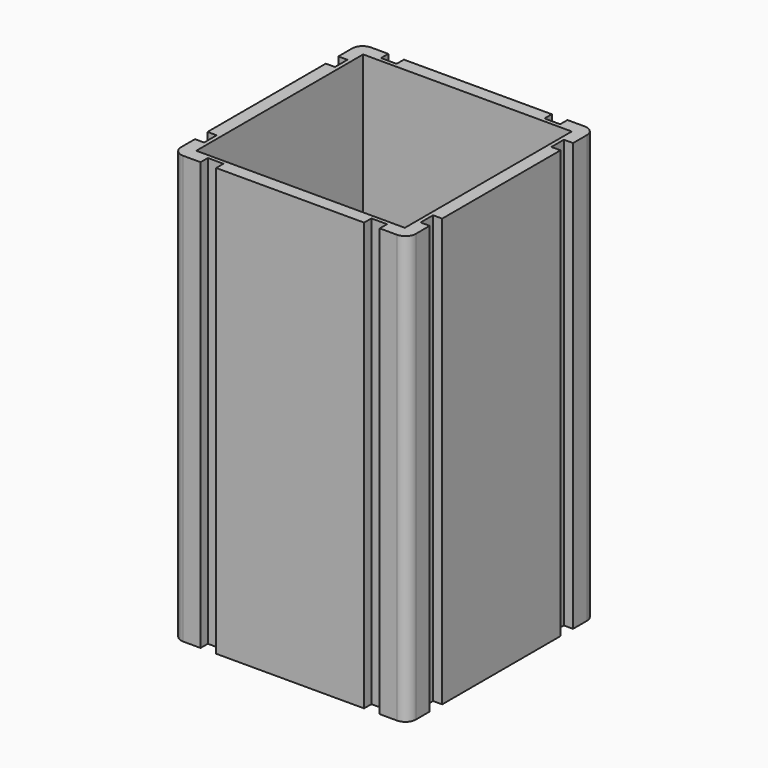
from build123d import *

# Parameters (mm, degrees)
F0_W            = 40
F0_H            = 40
F1_DEPTH        = 82
F2_W            = 3
F2_H            = 1.75
F3_DEPTH        = 82
F3_COPIES_COUNT = 4


# Not quite as in the source:
# - a pattern or mirror of a feature is missing from the dataset's text; its kind, count and spacing are read off the source's solid


with BuildPart() as f1:
    # F0 (on Top) → F1 (new body)
    with BuildSketch(Plane.XY):
        with BuildLine():
            Line((-20.5, -22.5), (20.5, -22.5))
            ThreePointArc((20.5, -22.5), (21.9142135624, -21.9142135624), (22.5, -20.5))
            Line((22.5, -20.5), (22.5, 20.5))
            ThreePointArc((22.5, 20.5), (21.9142135624, 21.9142135624), (20.5, 22.5))
            Line((20.5, 22.5), (-20.5, 22.5))
            ThreePointArc((-20.5, 22.5), (-21.9142135624, 21.9142135624), (-22.5, 20.5))
            Line((-22.5, 20.5), (-22.5, -20.5))
            ThreePointArc((-22.5, -20.5), (-21.9142135624, -21.9142135624), (-20.5, -22.5))
        make_face()
        Rectangle(F0_W, F0_H, mode=Mode.SUBTRACT)
    extrude(amount=F1_DEPTH)

    # F2 (on face) → F3 (cut, through all)
    with BuildSketch(Plane.XY.offset(82)):
        with Locations((-15.68, 21.625)):
            Rectangle(F2_W, F2_H)
        with Locations((15.68, 21.625)):
            Rectangle(F2_W, F2_H)
    f3 = extrude(amount=-F3_DEPTH, mode=Mode.SUBTRACT)

    # F3_copies: F3 ×4 about axis
    f3_copies_axis = Axis((0, 0, 0), (0, 0, 1))
    for i in range(1, F3_COPIES_COUNT):
        add(f3.rotate(f3_copies_axis, i * 360 / F3_COPIES_COUNT), mode=Mode.SUBTRACT)


solid = f1.part
